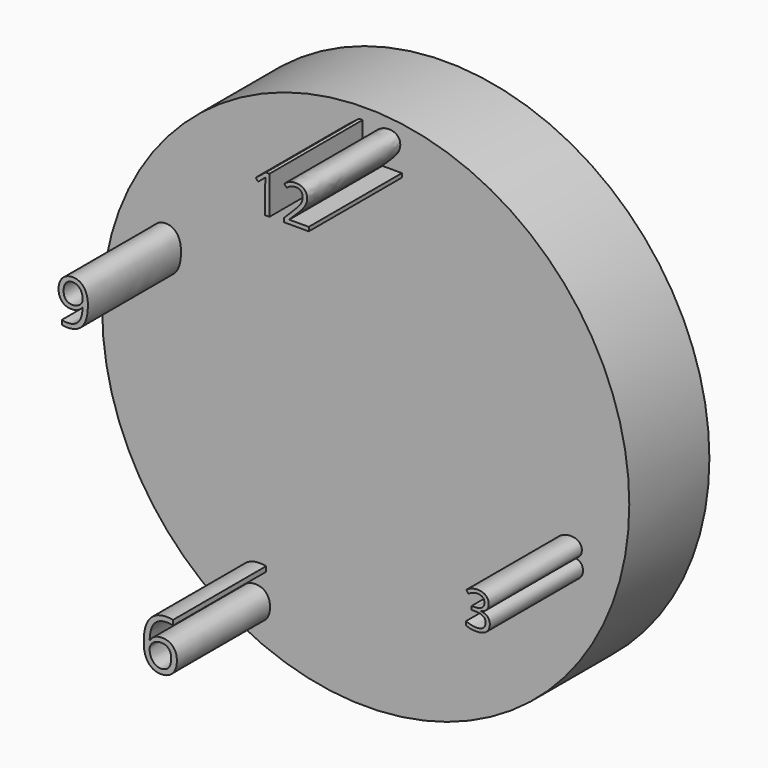
from build123d import *

# Parameters (mm, degrees)
F0_R         = 57.4992253997
F5_DEPTH     = 21.844
F4_TEXT_SIZE = 13.6931284538
F6_DEPTH     = 25.4
F2_TEXT_SIZE = 11.0598339234
F7_DEPTH     = 25.4
F3_TEXT_SIZE = 15.536431844
F8_DEPTH     = 25.4
F1_TEXT_SIZE = 11.5864910185
F9_DEPTH     = 25.4


# Not quite as in the source:
# - Text() gives the source's letters only with a copy of the font that has no kerning and outlines rounded to 1/6400 em; it was checked with that copy


with BuildPart() as f5:
    # F0 (on Front) → F5 (new body)
    with BuildSketch(Plane.XZ):
        with Locations((1.8959720619, 4.3607344851)):
            Circle(F0_R)
    extrude(amount=-F5_DEPTH)

    # F4 (on Front) → F6 (join)
    with BuildSketch(Plane.XZ):
        with Locations((-45.5033183098, 15.5469672754)):
            Text('9', F4_TEXT_SIZE, font='Open Sans', text_align=(TextAlign.LEFT, TextAlign.BOTTOM))
    extrude(amount=F6_DEPTH)

    # F2 (on Front) → F7 (join)
    with BuildSketch(Plane.XZ):
        with Locations((43.6073467135, -13.8405924663)):
            Text('3', F2_TEXT_SIZE, font='Open Sans', text_align=(TextAlign.LEFT, TextAlign.BOTTOM))
    extrude(amount=F7_DEPTH)

    # F3 (on Front) → F8 (join)
    with BuildSketch(Plane.XZ):
        with Locations((-27.1123927087, -44.3657338619)):
            Text('6', F3_TEXT_SIZE, font='Open Sans', text_align=(TextAlign.LEFT, TextAlign.BOTTOM))
    extrude(amount=F8_DEPTH)

    # F1 (on Front) → F9 (join)
    with BuildSketch(Plane.XZ):
        with Locations((-2.84395786, 51.0016344488)):
            Text('12', F1_TEXT_SIZE, font='Open Sans', text_align=(TextAlign.LEFT, TextAlign.BOTTOM))
    extrude(amount=F9_DEPTH)


solid = f5.part
